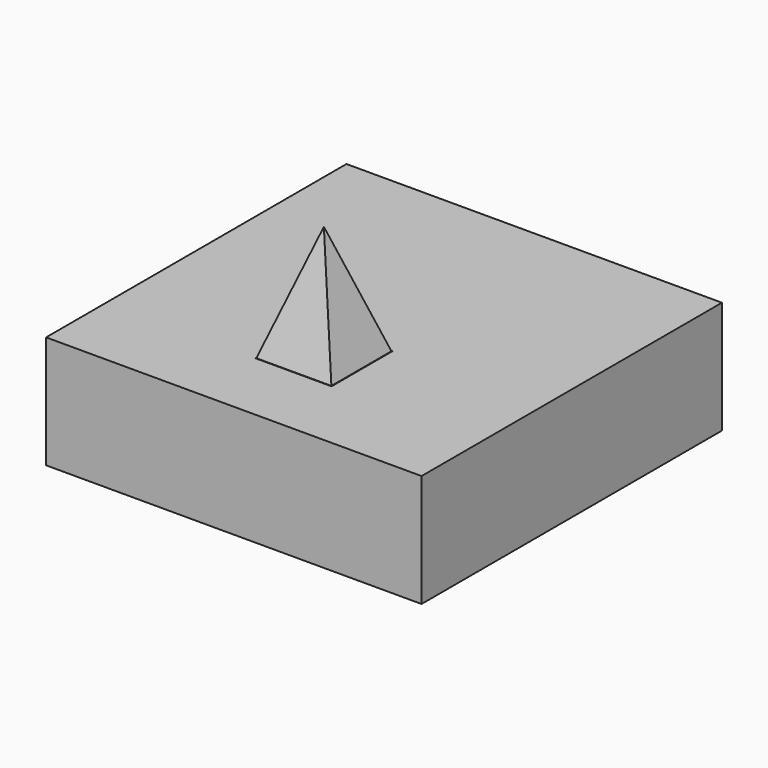
from build123d import *

# Parameters (mm, degrees)
F0_W     = 150
F0_H     = 150
F0_W_2   = 30.4
F0_H_2   = 30.4
F1_DEPTH = 45
F2_W     = 30
F2_H     = 30
F3_DEPTH = 45
F4_SIZE2 = 14.99999
F4_SIZE  = 44.99999


# Not quite as in the source:
# - a fillet or chamfer is up to 0.001 mm smaller than in the source, because OpenCascade refuses the exact size


with BuildPart() as f1:
    # F0 (on Top) → F1 (new body)
    with BuildSketch(Plane.XY):
        with Locations((-16.6580903113, -18.8472156852)):
            Rectangle(F0_W, F0_H)
        with Locations((-16.6580903113, -48.8472156852)):
            Rectangle(F0_W_2, F0_H_2, mode=Mode.SUBTRACT)
    extrude(amount=-F1_DEPTH)


with BuildPart() as f3:
    # F2 (on Top) → F3 (new body)
    with BuildSketch(Plane.XY):
        with Locations((-16.6773743331, -48.8492193)):
            Rectangle(F2_W, F2_H)
    extrude(amount=F3_DEPTH)

    # F4 (size 45 and 15 in the source; OpenCascade refuses exactly that, so slightly less here)
    f4_edges = [f3.edges().sort_by_distance(p)[0] for p in [
        (-1.677374, -48.849219, 45),
        (-16.677374, -33.849219, 45),
        (-31.677374, -48.849219, 45),
        (-16.677374, -63.849219, 45),
    ]]
    chamfer(f4_edges, length=F4_SIZE, length2=F4_SIZE2)


solid = Compound([f1.part, f3.part])
